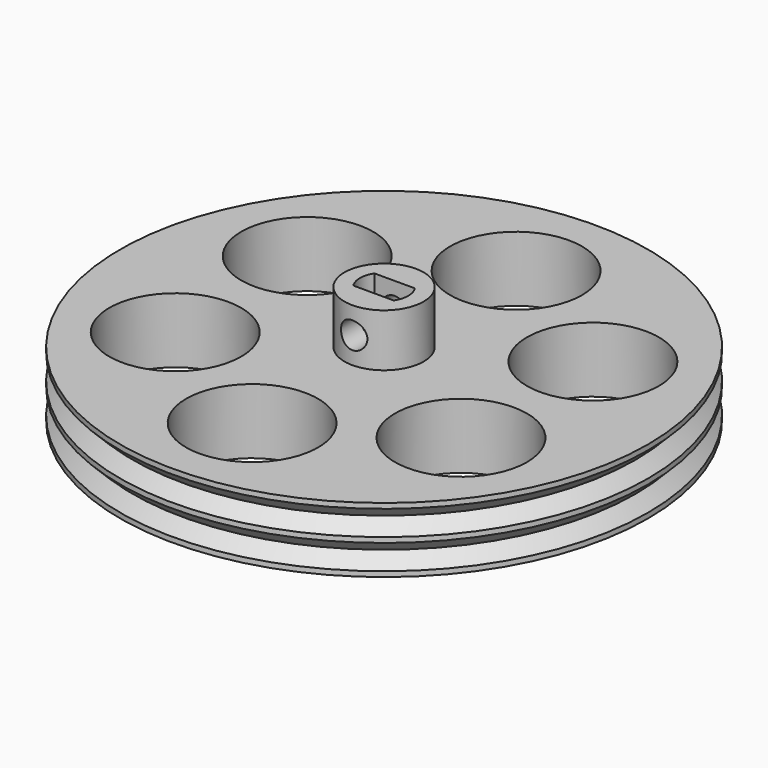
from build123d import *

# Parameters (mm, degrees)
F0_R             = 30
F0_R_2           = 4.5
F1_DEPTH         = 7.414
F2_DEPTH         = 6
F3_R             = 1.5
F4_DEPTH         = 12.5
F5_W             = 4.6
F5_H             = 3
F6_DEPTH         = 13.414
F9_R             = 7.5
F10_DEPTH        = 25
F10_COPIES_COUNT = 6


# Not quite as in the source:
# - a pattern or mirror of a feature is missing from the dataset's text; its kind, count and spacing are read off the source's solid


with BuildPart() as f1:
    # F0 (on Top) → F1 (new body)
    with BuildSketch(Plane.XY):
        Circle(F0_R)
        Circle(F0_R_2, mode=Mode.SUBTRACT)
        Circle(F0_R_2)
    extrude(amount=-F1_DEPTH)

    # F0 (on Top) → F2 (join)
    with BuildSketch(Plane.XY):
        Circle(F0_R_2)
    extrude(amount=F2_DEPTH)

    # F3 (on Front) → F4 (cut, symmetric)
    with BuildSketch(Plane.XZ):
        with Locations((0, 3)):
            Circle(F3_R)
    extrude(amount=F4_DEPTH, both=True, mode=Mode.SUBTRACT)

    # F5 (on face) → F6 (cut, through all)
    with BuildSketch(Plane.XY.offset(6)):
        Rectangle(F5_W, F5_H)
        with BuildLine():
            ThreePointArc((-2.3, 1.5), (-2.7459060435, 0), (-2.3, -1.5))
            Line((-2.3, -1.5), (-2.3, 1.5))
        make_face()
        with BuildLine():
            Line((2.3, 1.5), (2.3, -1.5))
            ThreePointArc((2.3, -1.5), (2.745183651, 0), (2.3, 1.5))
        make_face()
    extrude(amount=-F6_DEPTH, mode=Mode.SUBTRACT)

    # F7 (on Front) → F8 (revolve, cut)
    with BuildSketch(Plane.XZ):
        Polygon((30, -3.4142135624), (30, -0.5857864376), (28.5857864376, -2), align=None)
        Polygon((30, -6.8282135624), (30, -3.9997864376), (28.5857864376, -5.414), align=None)
    revolve(axis=Axis((0, 0, 0.7614716887), (0, 0, -1)), mode=Mode.SUBTRACT)

    # F9 (on face) → F10 (cut)
    with BuildSketch(Plane.XY):
        with Locations((0, 18.75)):
            Circle(F9_R)
    f10 = extrude(amount=-F10_DEPTH, mode=Mode.SUBTRACT)

    # F10_copies: F10 ×6 about axis
    f10_copies_axis = Axis((0, 0, 0), (0, 0, 1))
    for i in range(1, F10_COPIES_COUNT):
        add(f10.rotate(f10_copies_axis, i * 360 / F10_COPIES_COUNT), mode=Mode.SUBTRACT)


solid = f1.part
